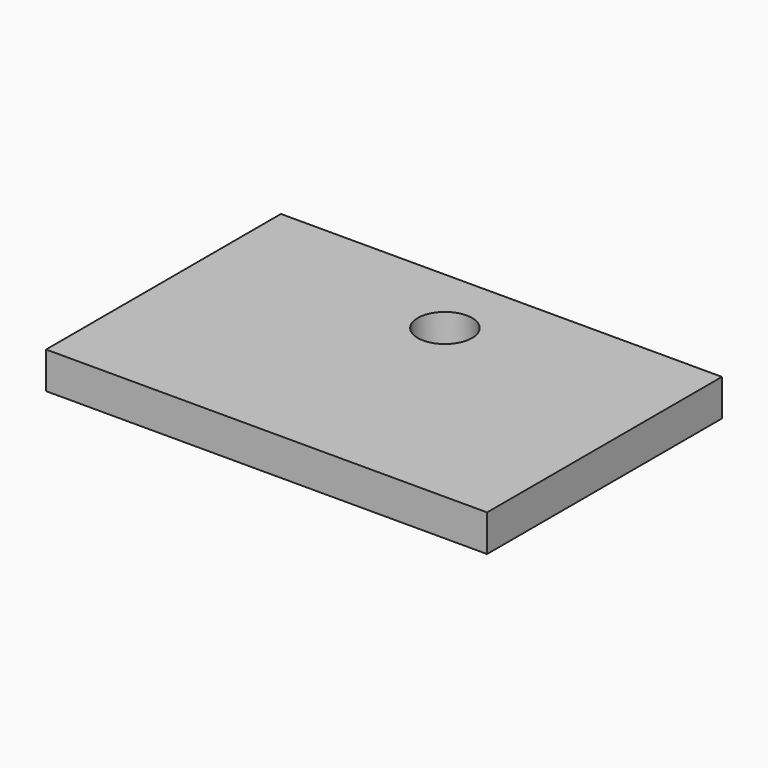
from build123d import *

# Parameters (mm, degrees)
F0_W          = 76.319962422
F0_H          = 50.8
F1_DEPTH      = 6.35
F2_R          = 4.7045967167
F3_DEPTH      = 99
F3_DEPTH_BACK = 6.351


# Not quite as in the source:
# - an extrude ends at something that could not be found from the text; its depth is read off the source's solid
# - a feature names something its author has since deleted; it is built from what else it names


with BuildPart() as f1:
    # F0 (on Top) → F1 (new body)
    with BuildSketch(Plane.XY):
        with Locations((4.271581769, -3.4901092946)):
            Rectangle(F0_W, F0_H)
    extrude(amount=F1_DEPTH)

    # F2 (on face) → F3 (cut, two sides)
    with BuildSketch(Plane.XY.offset(6.35)) as f3_sk:
        with Locations((4.271581769, 9.693203494)):
            Circle(F2_R)
    extrude(amount=F3_DEPTH, mode=Mode.SUBTRACT)
    extrude(f3_sk.sketch, amount=-F3_DEPTH_BACK, mode=Mode.SUBTRACT)


solid = f1.part
